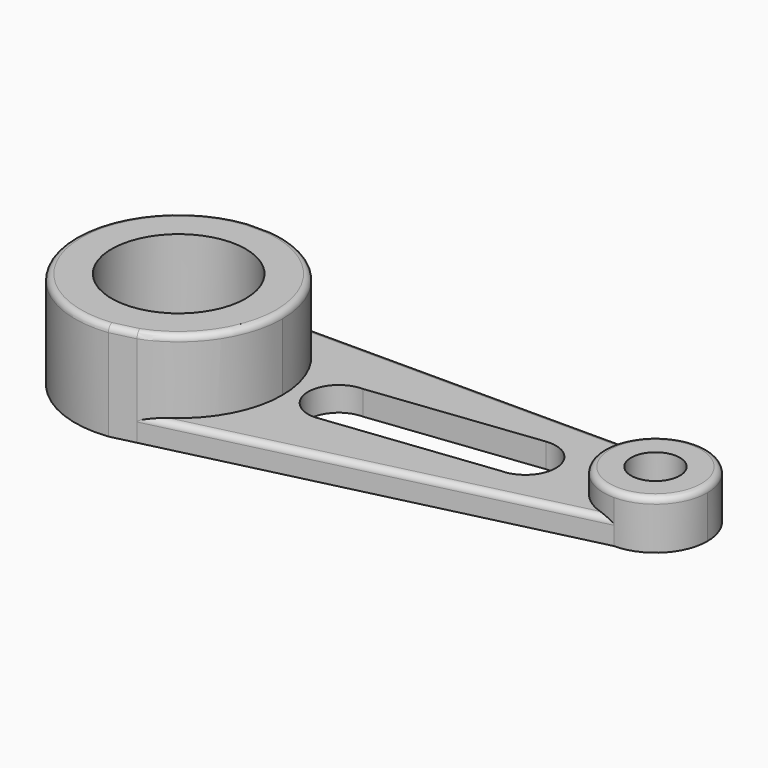
from build123d import *

# Parameters (mm, degrees)
F0_R          = 34.925
F1_DEPTH      = 50.8
F0_R_2        = 12.7
F2_DEPTH      = 25.4
F3_DEPTH      = 12.7
F4_T1_DEPTH   = 39.8737412721
F4_T3_DEPTH   = 39.5290127835
F4_T6_ANGLE   = 196.8788005765
F4_T8_ANGLE   = 169.8162488072
F4_3_T1_DEPTH = 273.9624836944
F4_3_T3_DEPTH = 277.6947318263


# Not quite as in the source:
# - a fillet or chamfer that OpenCascade refuses, or shapes differently, is made with other operations: its cross-section is extruded or revolved along the edge and cut away or added


with BuildPart() as f1:
    # F0 (on Top) → F1 (new body)
    with BuildSketch(Plane.XY):
        with BuildLine():
            ThreePointArc((-173.0769900862, -26.5584976592), (-186.7297586174, 9.3221137399), (-220.7812336944, 27.051))
            Line((-220.7812336944, 27.051), (-233.3227464779, 27.051))
            ThreePointArc((-233.3227464779, 27.051), (-280.6614877454, -32.829254051), (-220.7812336944, -80.1679953185))
            Line((-220.7812336944, -80.1679953185), (-208.2524858785, -77.1537471057))
            ThreePointArc((-208.2524858785, -77.1537471057), (-182.7349286729, -57.3691888669), (-173.0769900862, -26.5584976592))
        make_face()
        with Locations((-227.0519900862, -26.5584976592)):
            Circle(F0_R, mode=Mode.SUBTRACT)
    extrude(amount=F1_DEPTH)

    # F4: fillet of radius 3.175 on 4 edges, made by hand

    # F4_s2 → F4_t1 (cut)
    with BuildSketch(Plane(origin=(-240.0526530104, -57.7534396052, 0), x_dir=(0, 0, 1), z_dir=(0.97225774, 0.2339121354, 0))):
        with BuildLine():
            ThreePointArc((50.8, 23.1255441239), (49.8700640303, 25.3706081542), (47.625, 26.3005441239))
            Line((47.625, 26.3005441239), (50.8, 26.3005441239))
            Line((50.8, 26.3005441239), (50.8, 23.1255441239))
        make_face()
    extrude(amount=F4_T1_DEPTH, mode=Mode.SUBTRACT)

    # F4_s4 → F4_t3 (cut)
    with BuildSketch(Plane.YZ.offset(-246.8164964779)):
        with BuildLine():
            ThreePointArc((27.051, 47.625), (26.1210640303, 49.8700640303), (23.876, 50.8))
            Line((23.876, 50.8), (27.051, 50.8))
            Line((27.051, 50.8), (27.051, 47.625))
        make_face()
    extrude(amount=F4_T3_DEPTH, mode=Mode.SUBTRACT)

    # F4_s5 → F4_t6 (revolve, cut)
    with BuildSketch(Plane(origin=(-226.0170180044, 6.9756210319, 0), x_dir=(0, 0, 1), z_dir=(0.9995240697, -0.030848567, 0))):
        with BuildLine():
            ThreePointArc((47.625, -20.4249138064), (49.8700640303, -19.4949778367), (50.8, -17.2499138064))
            Line((50.8, -17.2499138064), (50.8, -20.4249138064))
            Line((50.8, -20.4249138064), (47.625, -20.4249138064))
        make_face()
    revolve(axis=Axis((-227.0519900862, -26.5584976592, 50.8), (0, 0, 1)), revolution_arc=F4_T6_ANGLE, mode=Mode.SUBTRACT)

    # F4_s7 → F4_t8 (revolve, cut)
    with BuildSketch(Plane(origin=(-227.653997391, -7.0111486331, 0), x_dir=(0, 0, 1), z_dir=(-0.9995260975, -0.0307827937, 0))):
        with BuildLine():
            ThreePointArc((47.625, 34.4183830445), (49.8700640303, 33.4884470747), (50.8, 31.2433830445))
            Line((50.8, 31.2433830445), (50.8, 34.4183830445))
            Line((50.8, 34.4183830445), (47.625, 34.4183830445))
        make_face()
    revolve(axis=Axis((-227.0519900862, -26.5584976592, 50.8), (0, 0, -1)), revolution_arc=F4_T8_ANGLE, mode=Mode.SUBTRACT)


with BuildPart() as f2:
    # F0 (on Top) → F2 (new body)
    with BuildSketch(Plane.XY):
        with BuildLine():
            ThreePointArc((0, -27.051), (19.1279455379, -19.1279455379), (27.051, 0))
            ThreePointArc((27.051, 0), (19.1279455379, 19.1279455379), (0, 27.051))
            ThreePointArc((0, 27.051), (-27.051, 0), (0, -27.051))
        make_face()
        Circle(F0_R_2, mode=Mode.SUBTRACT)
    extrude(amount=F2_DEPTH)

    # F4#2: fillet of radius 3.175 on 1 edges, made by hand

    # F4_2_s1 → F4_2_t2 (revolve, cut)
    with BuildSketch(Plane.YZ):
        with BuildLine():
            ThreePointArc((27.051, 22.225), (26.1210640303, 24.4700640303), (23.876, 25.4))
            Line((23.876, 25.4), (27.051, 25.4))
            Line((27.051, 25.4), (27.051, 22.225))
        make_face()
    revolve(axis=Axis((0, 0, 25.4), (0, 0, -1)), mode=Mode.SUBTRACT)


with BuildPart() as f3:
    # F0 (on Top) → F3 (new body)
    with BuildSketch(Plane.XY):
        with BuildLine():
            ThreePointArc((0, -27.051), (-27.051, 0), (0, 27.051))
            Line((0, 27.051), (-220.7812336944, 27.051))
            ThreePointArc((-220.7812336944, 27.051), (-186.7297586174, 9.3221137399), (-173.0769900862, -26.5584976592))
            ThreePointArc((-173.0769900862, -26.5584976592), (-182.7349286729, -57.3691888669), (-208.2524858785, -77.1537471057))
            Line((-208.2524858785, -77.1537471057), (0, -27.051))
        make_face()
        with BuildLine():
            ThreePointArc((-150.8519900862, -33.5203076851), (-166.7269900862, -17.6453076851), (-150.8519900862, -1.7703076851))
            Line((-150.8519900862, -1.7703076851), (-63.8156668227, 8.5186394182))
            ThreePointArc((-63.8156668227, 8.5186394182), (-46.1044574819, -6.3131325916), (-61.9519900862, -23.1215860487))
            Line((-61.9519900862, -23.1215860487), (-150.8519900862, -33.5203076851))
        make_face(mode=Mode.SUBTRACT)
    extrude(amount=F3_DEPTH)

    # F4#3: fillet of radius 3.175 on 2 edges, made by hand

    # F4_3_s2 → F4_3_t1 (cut)
    with BuildSketch(Plane.YZ.offset(-260.4687336944)):
        with BuildLine():
            ThreePointArc((23.876, 12.7), (26.1210640303, 11.7700640303), (27.051, 9.525))
            Line((27.051, 9.525), (27.051, 12.7))
            Line((27.051, 12.7), (23.876, 12.7))
        make_face()
    extrude(amount=F4_3_T1_DEPTH, mode=Mode.SUBTRACT)

    # F4_3_s4 → F4_3_t3 (cut)
    with BuildSketch(Plane(origin=(-252.9909813708, -60.8662273882, 0), x_dir=(0, 0, 1), z_dir=(0.97225774, 0.2339121354, 0))):
        with BuildLine():
            ThreePointArc((9.525, 26.3005441239), (11.7700640303, 25.3706081542), (12.7, 23.1255441239))
            Line((12.7, 23.1255441239), (12.7, 26.3005441239))
            Line((12.7, 26.3005441239), (9.525, 26.3005441239))
        make_face()
    extrude(amount=F4_3_T3_DEPTH, mode=Mode.SUBTRACT)


solid = Compound([f1.part, f2.part, f3.part])
